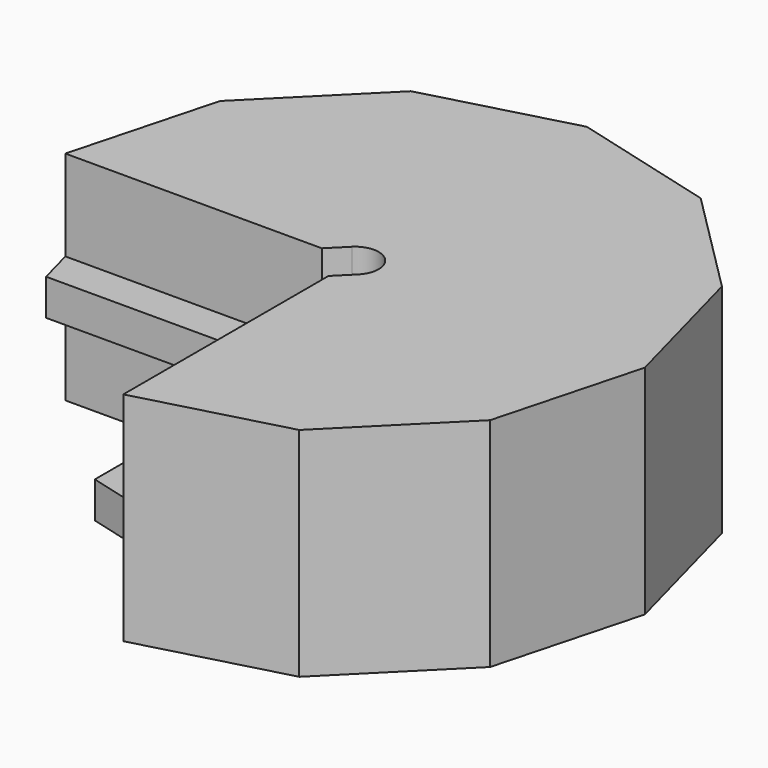
from build123d import *

# Parameters (mm, degrees)
F1_DEPTH  = 38.1
F2_W      = 50.8
F2_H      = 3.175
F3_DEPTH  = 6.35
F5_DEPTH  = 25.4
F6_W      = 44.45
F6_H      = 6.35
F7_DEPTH  = 6.35
F9_DEPTH  = 25.4
F10_R     = 4.1275
F11_DEPTH = 127
F13_DEPTH = 127


# Not quite as in the source:
# - a feature names something its author has since deleted; it is built from what else it names


with BuildPart() as f1:
    # F0 (on Top) → F1 (new body)
    with BuildSketch(Plane.XY):
        Polygon((43.9940905122, -25.4), (50.8, 0), (43.9940905122, 25.4), (25.4, 43.9940905122), (0, 50.8), (-25.4, 43.9940905122), (-43.9940905122, 25.4), (-50.8, 0), (0, 0), (0, -50.8), (25.4, -43.9940905122), align=None)
    extrude(amount=F1_DEPTH)

    # F2 (on face) → F3 (join)
    with BuildSketch(Plane.XZ):
        with Locations((-25.4, 20.6375)):
            Rectangle(F2_W, F2_H)
        with Locations((-25.4, 17.4625)):
            Rectangle(F2_W, F2_H)
    extrude(amount=F3_DEPTH)

    # F4 (on face) → F5 (cut)
    with BuildSketch(Plane.XY.offset(22.225)):
        Polygon((-49.0985226281, -6.35), (-50.8, 0), (-50.8, -6.35), align=None)
    extrude(amount=-F5_DEPTH, mode=Mode.SUBTRACT)

    # F6 (on face) → F7 (join)
    with BuildSketch(Plane(origin=(0, 0, 0), x_dir=(0, -1, 0), z_dir=(-1, 0, 0))):
        with Locations((28.575, 19.05)):
            Rectangle(F6_W, F6_H)
    extrude(amount=F7_DEPTH)

    # F8 (on face) → F9 (cut)
    with BuildSketch(Plane.XY.offset(22.225)):
        Polygon((-6.35, -50.8), (0, -50.8), (-6.35, -49.0985226281), align=None)
    extrude(amount=-F9_DEPTH, mode=Mode.SUBTRACT)

    # F10 (on face) → F11 (cut)
    with BuildSketch(Plane.XY.offset(38.1)):
        Circle(F10_R)
    extrude(amount=-F11_DEPTH, mode=Mode.SUBTRACT)

    # F12 (on face) → F13 (cut)
    with BuildSketch(Plane.XY.offset(38.1)):
        with BuildLine():
            ThreePointArc((-4.1275, 0), (-3.8133127704, 1.5795258671), (-2.9185832393, 2.9185832393))
            Line((-2.9185832393, 2.9185832393), (-5.8371664787, 0))
            Line((-5.8371664787, 0), (-4.1275, 0))
        make_face()
        with BuildLine():
            ThreePointArc((4.1275, 0), (1.5795258671, 3.8133127704), (-2.9185832393, 2.9185832393))
            ThreePointArc((-2.9185832393, 2.9185832393), (-3.8133127704, 1.5795258671), (-4.1275, 0))
            Line((-4.1275, 0), (-5.8371664787, 0))
            Line((-5.8371664787, 0), (-18.7979032201, -12.9607367414))
            Line((-18.7979032201, -12.9607367414), (-12.9607367414, -18.7979032201))
            Line((-12.9607367414, -18.7979032201), (0, -5.8371664787))
            Line((0, -5.8371664787), (0, -4.1275))
            ThreePointArc((0, -4.1275), (1.5795258671, -3.8133127704), (2.9185832393, -2.9185832393))
            ThreePointArc((2.9185832393, -2.9185832393), (3.8133127704, -1.5795258671), (4.1275, 0))
        make_face()
        with BuildLine():
            Line((0, -5.8371664787), (2.9185832393, -2.9185832393))
            ThreePointArc((2.9185832393, -2.9185832393), (1.5795258671, -3.8133127704), (0, -4.1275))
            Line((0, -4.1275), (0, -5.8371664787))
        make_face()
    extrude(amount=-F13_DEPTH, mode=Mode.SUBTRACT)


solid = f1.part
